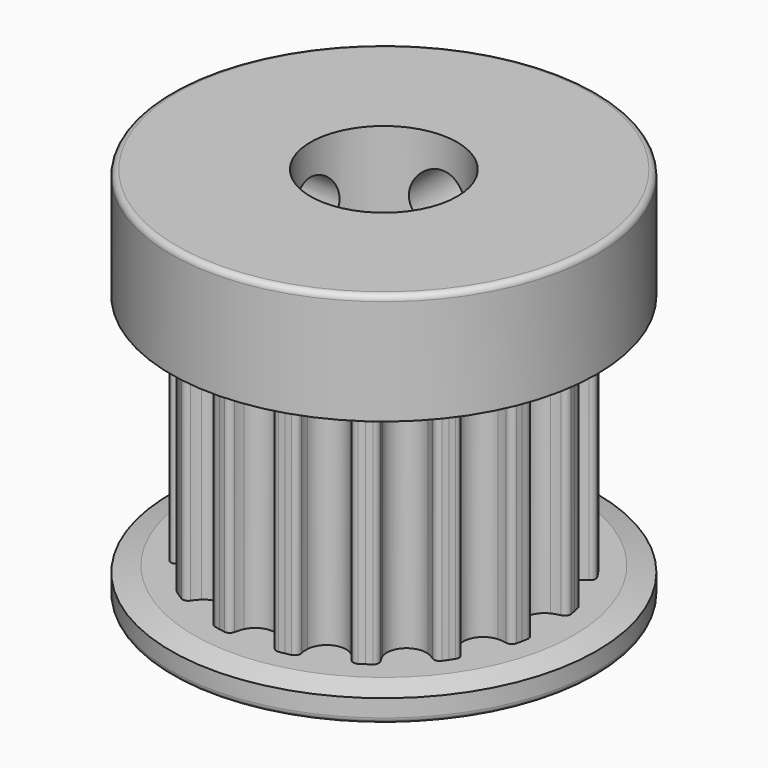
from build123d import *

# Parameters (mm, degrees)
F3_DEPTH    = 5
F4_COUNT    = 16
F5_R        = 9.2075
F6_DEPTH    = 1.27
F7_R        = 9.2075
F8_DEPTH    = 1.27
F9_R        = 9.2075
F10_DEPTH   = 3.81
F11_R       = 3.175
F12_DEPTH   = 16.351
F13_R       = 1.25
F14_DEPTH   = 9.2085
F15_R       = 1.25
F16_DEPTH   = 9.2085001
F17_SIZE2   = 0.2679491924
F17_SIZE    = 1
F17_2_SIZE2 = 0.2679491924
F17_2_SIZE  = 1
F18_R       = 0.25


# Not quite as in the source:
# - a feature names something its author has since deleted; it is built from what else it names


with BuildPart() as f3:
    # F2 (on Top) → F3 (new body, symmetric)
    with BuildSketch(Plane.XY):
        with BuildLine():
            ThreePointArc((0.7729699653, 6.6005393756), (0.459324865, 6.2389106877), (0, 6.1041174189))
            ThreePointArc((0, 6.1041174189), (-0.459324865, 6.2389106877), (-0.7729699653, 6.6005393756))
            ThreePointArc((-0.7729699653, 6.6005393756), (-0.840847916, 6.777273601), (-0.8862292653, 6.9610749495))
            ThreePointArc((-0.8862292653, 6.9610749495), (-0.9880853916, 7.1206605485), (-1.1725886371, 7.1630962207))
            ThreePointArc((-1.1725886371, 7.1630962207), (-1.2945077953, 7.1420698083), (-1.416050864, 7.1189684316))
            Line((-1.416050864, 7.1189684316), (0, 0))
            Line((0, 0), (1.416050864, 7.1189684316))
            ThreePointArc((1.416050864, 7.1189684316), (1.2945077953, 7.1420698083), (1.1725886371, 7.1630962207))
            ThreePointArc((1.1725886371, 7.1630962207), (0.9880853916, 7.1206605485), (0.8862292653, 6.9610749495))
            ThreePointArc((0.8862292653, 6.9610749495), (0.840847916, 6.777273601), (0.7729699653, 6.6005393756))
        make_face()
    extrude(amount=F3_DEPTH, both=True)

    # F4: F3 ×16 about axis
    f4_axis = Axis((0, 0, 0), (0, 0, -1))


with BuildPart() as f3_1:
    add(f3.part)
    for i in range(1, F4_COUNT):
        add(f3.part.rotate(f4_axis, i * 360 / F4_COUNT))

    # F5 (on face) → F6 (join)
    with BuildSketch(Plane(origin=(0, 0, -5), x_dir=(1, 0, 0), z_dir=(0, 0, -1))):
        Circle(F5_R)
    extrude(amount=F6_DEPTH)

    # F7 (on face) → F8 (join)
    with BuildSketch(Plane.XY.offset(5)):
        Circle(F7_R)
    extrude(amount=F8_DEPTH)

    # F9 (on face) → F10 (join)
    with BuildSketch(Plane.XY.offset(6.27)):
        Circle(F9_R)
    extrude(amount=F10_DEPTH)

    # F11 (on face) → F12 (cut, through all)
    with BuildSketch(Plane.XY.offset(10.08)):
        Circle(F11_R)
    extrude(amount=-F12_DEPTH, mode=Mode.SUBTRACT)

    # F13 (on Front) → F14 (cut, through all)
    with BuildSketch(Plane.XZ):
        with Locations((0, 7.5)):
            Circle(F13_R)
    extrude(amount=-F14_DEPTH, mode=Mode.SUBTRACT)

    # F15 (on Right) → F16 (cut, through all)
    with BuildSketch(Plane.YZ):
        with Locations((0, 7.5)):
            Circle(F15_R)
    extrude(amount=-F16_DEPTH, mode=Mode.SUBTRACT)

    # F17
    f17_edges = [f3_1.edges().sort_by_distance(p)[0] for p in [
        (-9.2075, 0, -5),
    ]]
    f17_side = f3_1.faces().sort_by_distance((-8.947073, 0, -5))[0]
    chamfer(f17_edges, length=F17_SIZE, length2=F17_SIZE2, reference=f17_side)

    # F17#2
    f17_2_edges = [f3_1.edges().sort_by_distance(p)[0] for p in [
        (-9.2075, 0, 5),
    ]]
    f17_2_side = f3_1.faces().sort_by_distance((-8.947073, 0, 5))[0]
    chamfer(f17_2_edges, length=F17_2_SIZE, length2=F17_2_SIZE2, reference=f17_2_side)

    # F18
    f18_edges = [f3_1.edges().sort_by_distance(p)[0] for p in [
        (-9.2075, 0, 10.08),
        (-9.2075, 0, -6.27),
    ]]
    fillet(f18_edges, radius=F18_R)


solid = f3_1.part
